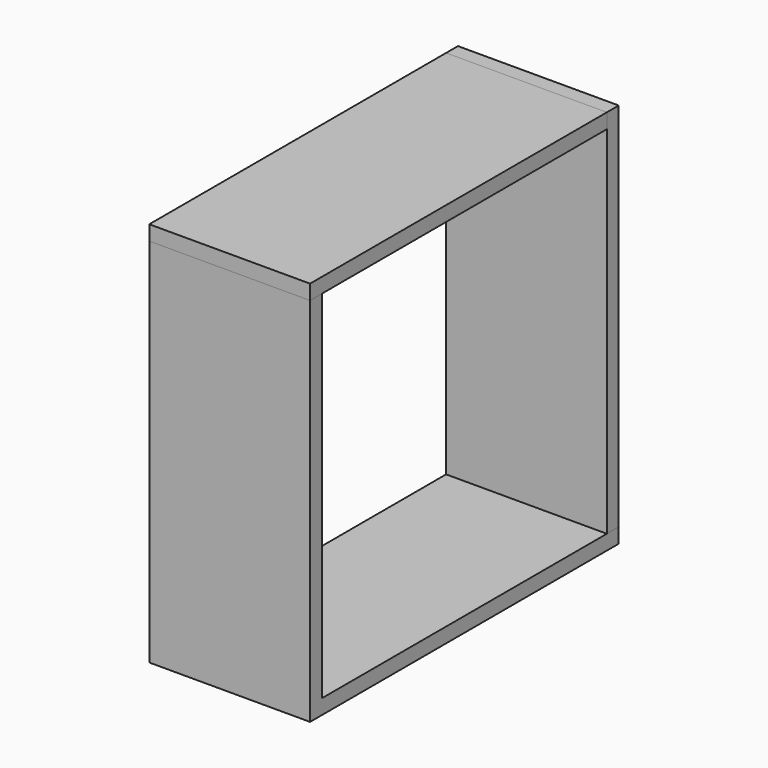
from build123d import *

# Parameters (mm, degrees)
F0_W     = 130
F0_H     = 12
F1_DEPTH = 300
F2_W     = 130
F2_H     = 12
F3_DEPTH = 300
F4_W     = 130
F4_H     = 312
F5_DEPTH = 12


with BuildPart() as f1:
    # F0 (on Top) → F1 (new body)
    with BuildSketch(Plane.XY):
        with Locations((-872.942913402, -1763.4354934643)):
            Rectangle(F0_W, F0_H)
    extrude(amount=F1_DEPTH)

    # F4 (on face) → F5 (join)
    with BuildSketch(Plane(origin=(0, 0, 0), x_dir=(1, 0, 0), z_dir=(0, 0, -1))):
        with Locations((-872.942913402, 1613.4354934643)):
            Rectangle(F4_W, F4_H)
    extrude(amount=F5_DEPTH)


with BuildPart() as f1b:
    # F0 (on Top) → F1, piece 2 (new body)
    with BuildSketch(Plane.XY):
        with Locations((-872.942913402, -1463.4354934643)):
            Rectangle(F0_W, F0_H)
    extrude(amount=F1_DEPTH)


with BuildPart() as f3:
    # F2 (on face) → F3 (new body)
    with BuildSketch(Plane.XZ.offset(1469.4354934643)):
        with Locations((-872.942913402, 294)):
            Rectangle(F2_W, F2_H)
    extrude(amount=F3_DEPTH)


solid = Compound([f1.part, f1b.part, f3.part])
